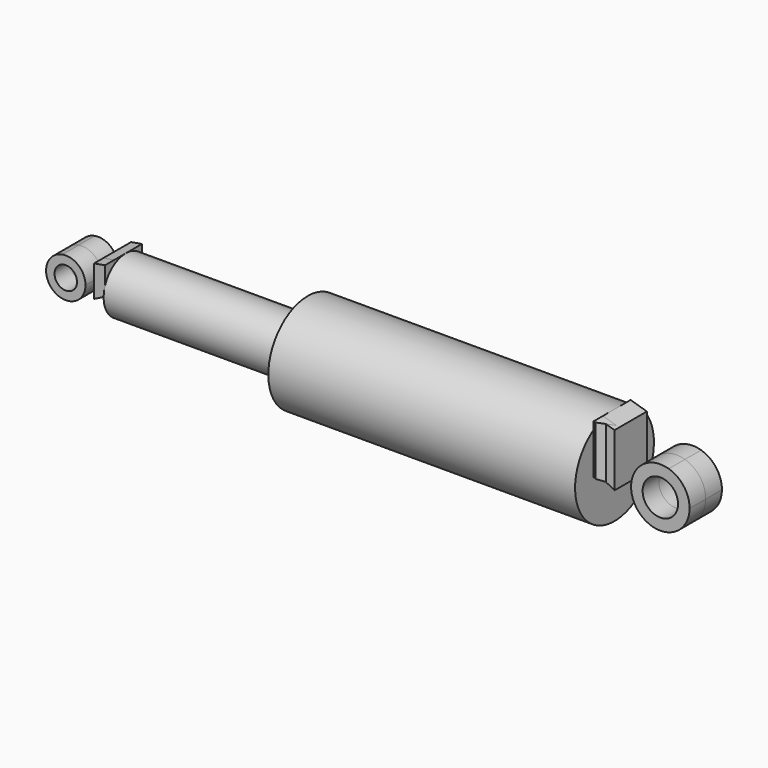
from build123d import *

# Parameters (mm, degrees)
F3_DEPTH    = 7
F0_R        = 3.8878640564
F0_R_2      = 6.1424275905
F4_DEPTH    = 2
F5_T1_DEPTH = 44.0991409969


# Not quite as in the source:
# - a fillet or chamfer that OpenCascade refuses, or shapes differently, is made with other operations: its cross-section is extruded or revolved along the edge and cut away or added


with BuildPart() as f1:
    # F0 (on Front) → F1 (revolve)
    with BuildSketch(Plane.XZ):
        Polygon((-25.0066287739, 17.072636364), (-25.0066287739, 9.5776912849), (67.6134303212, 9.5776912849), (74.2266178131, 9.5776912849), (74.2266178131, 0), (81.2806785107, 0), (81.2806785107, 17.072636364), align=None)
    revolve(axis=Axis((-10.2194553203, 0, 0), (-1, 0, 0)))


with BuildPart() as f2:
    # F0 (on Front) → F2 (revolve)
    with BuildSketch(Plane.XZ):
        Polygon((-88.0523409618, 9.5776912849), (-88.0523409618, 0), (67.6134303212, 0), (67.6134303212, 9.5776912849), (-25.0066287739, 9.5776912849), align=None)
    revolve(axis=Axis((-10.2194553203, 0, 0), (-1, 0, 0)))

    # F0 (on Front) → F3 (join, symmetric)
    with BuildSketch(Plane.XZ):
        Polygon((-91.8371824493, -1.9084735904), (-88.0523409618, 0), (-88.0523409618, 9.5776912849), (-91.8371824493, 8.9197958771), align=None)
    extrude(amount=F3_DEPTH, both=True)


with BuildPart() as f3:
    # F0 (on Front) → F3, piece 2 (new body, symmetric)
    with BuildSketch(Plane.XZ):
        with BuildLine():
            ThreePointArc((-104.4060712545, 6.7350242686), (-109.725277002, -2.1475884562), (-100.1575113171, -6.1039274712))
            ThreePointArc((-100.1575113171, -6.1039274712), (-97.4142233615, -3.5840521197), (-96.3993484931, 0))
            ThreePointArc((-96.3993484931, 0), (-98.8349018086, 5.2313516723), (-104.4060712545, 6.7350242686))
        make_face()
        with Locations((-103.2353639603, 0)):
            Circle(F0_R, mode=Mode.SUBTRACT)
    extrude(amount=F3_DEPTH, both=True)


with BuildPart() as f3b:
    # F0 (on Front) → F3, piece 3 (new body, symmetric)
    with BuildSketch(Plane.XZ):
        Polygon((86.8883872816, 15.3799332838), (81.2806785107, 17.072636364), (81.2806785107, 0), (86.8883872816, -3.0023778334), align=None)
    extrude(amount=F3_DEPTH, both=True)


with BuildPart() as f3c:
    # F0 (on Front) → F3, piece 4 (new body, symmetric)
    with BuildSketch(Plane.XZ):
        with BuildLine():
            ThreePointArc((112.8962301513, 0), (110.8970724106, 6.0445930034), (105.6880680425, 9.7051953777))
            ThreePointArc((105.6880680425, 9.7051953777), (93.3911995488, 3.8763654791), (97.9734557929, -8.9373443838))
            ThreePointArc((97.9734557929, -8.9373443838), (107.9673365894, -8.6972024121), (112.8962301513, 0))
        make_face()
        with Locations((102.7585268021, 0)):
            Circle(F0_R_2, mode=Mode.SUBTRACT)
    extrude(amount=F3_DEPTH, both=True)


with BuildPart() as f4:
    # F4 (new, symmetric): a face of the model
    f4_faces = [f3b.part.faces().sort_by_distance(p)[0] for p in [
        (84.1190568725, -7, 7.3480952717),
    ]]
    extrude(f4_faces, amount=F4_DEPTH, both=True)

    # F5: chamfer of 5 on 1 edges, made by hand

    # F5_s2 → F5_t1 (cut)
    with BuildSketch(Plane.XY.offset(-15.8607927732)):
        Polygon((86.8883872816, -4), (81.8883872816, -9), (86.8883872816, -9), align=None)
    extrude(amount=F5_T1_DEPTH, mode=Mode.SUBTRACT)


with BuildPart() as f4b:
    # F4#2 (new, symmetric): a face of the model
    f4_2_faces = [f2.part.faces().sort_by_distance(p)[0] for p in [
        (-89.9834206726, -7, 4.1341467443),
    ]]
    extrude(f4_2_faces, amount=F4_DEPTH, both=True)


solid = Compound([f1.part, f2.part, f3.part, f3b.part, f3c.part, f4.part, f4b.part])
